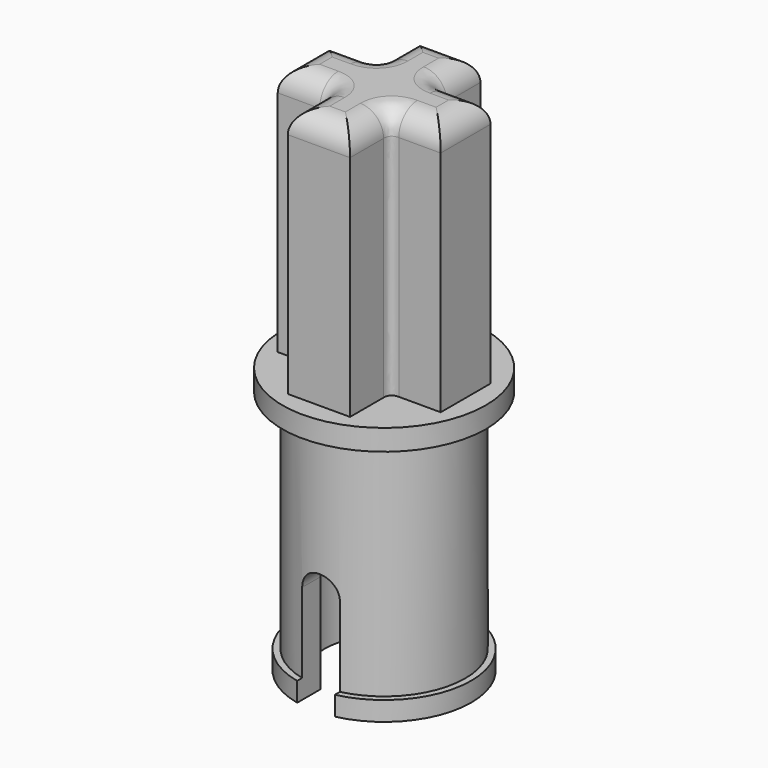
from build123d import *

# Parameters (mm, degrees)
F0_R         = 2.3495
F1_DEPTH     = 15.6718
F3_R         = 2.5273
F4_DEPTH     = 0.5588
F5_DEPTH     = 12.7
F6_R         = 2.9464
F7_DEPTH     = 8.5598
F8_R         = 12.7
F9_DEPTH     = 7.9502
F10_W        = 1.4605
F10_H        = 1.8034
F10_W_2      = 1.8034
F10_H_2      = 1.4605
F11_DEPTH    = 7.2898
F12_T1_DEPTH = 7.9030102448
F13_R        = 0.6745312693
F14_R        = 1.7145
F15_DEPTH    = 5.8674


# Not quite as in the source:
# - a fillet or chamfer that OpenCascade refuses, or shapes differently, is made with other operations: its cross-section is extruded or revolved along the edge and cut away or added


with BuildPart() as f1:
    # F0 (on Top) → F1 (new body)
    with BuildSketch(Plane.XY):
        Circle(F0_R)
    extrude(amount=F1_DEPTH)

    # F3 (on face) → F4 (join)
    with BuildSketch(Plane(origin=(0, 0, 0), x_dir=(1, 0, 0), z_dir=(0, 0, -1))):
        Circle(F3_R)
    extrude(amount=-F4_DEPTH)

    # F2 (on Front) → F5 (cut, symmetric)
    with BuildSketch(Plane.XZ):
        with BuildLine():
            Line((-0.5461, -2.8702), (0.5461, -2.8702))
            Line((0.5461, -2.8702), (0.5461, 2.8702))
            ThreePointArc((0.5461, 2.8702), (0, 2.3241), (-0.5461, 2.8702))
            Line((-0.5461, 2.8702), (-0.5461, -2.8702))
        make_face()
        with BuildLine():
            ThreePointArc((-0.5461, 2.8702), (0, 2.3241), (0.5461, 2.8702))
            Line((0.5461, 2.8702), (-0.5461, 2.8702))
        make_face()
        with BuildLine():
            Line((-0.5461, 2.8702), (0.5461, 2.8702))
            ThreePointArc((0.5461, 2.8702), (0, 3.4163), (-0.5461, 2.8702))
        make_face()
    extrude(amount=F5_DEPTH, both=True, mode=Mode.SUBTRACT)

    # F6 (on face) → F7 (join)
    with BuildSketch(Plane.XY.offset(15.6718)):
        Circle(F6_R)
    extrude(amount=-F7_DEPTH)

    # F8 (on face) → F9 (cut)
    with BuildSketch(Plane.XY.offset(15.6718)):
        Circle(F8_R)
    extrude(amount=-F9_DEPTH, mode=Mode.SUBTRACT)

    # F10 (on face) → F11 (join)
    with BuildSketch(Plane.XY.offset(7.7216)):
        with Locations((1.63195, 0)):
            Rectangle(F10_W, F10_H)
        with Locations((0, -1.63195)):
            Rectangle(F10_W_2, F10_H_2)
        Rectangle(F10_W_2, F10_H)
        with Locations((-1.63195, 0)):
            Rectangle(F10_W, F10_H)
        with Locations((0, 1.63195)):
            Rectangle(F10_W_2, F10_H_2)
    extrude(amount=F11_DEPTH)

    # F12: fillet of radius 0.2452840979 on 4 edges, made by hand

    # F12_s2 → F12_t1 (join)
    with BuildSketch(Plane.XY.offset(7.1083897552)):
        with BuildLine():
            add(Edge.make_bspline(
                [(-1.1469840979, -0.9017), (-0.9017, -0.9017), (-0.9017, -1.1469840979)],
                knots=[0, 0, 0, 1, 1, 1], degree=2, weights=[1, 1, 1]))
            Line((-0.9017, -1.1469840979), (-0.9017, -0.9017))
            Line((-0.9017, -0.9017), (-1.1469840979, -0.9017))
        make_face()
        with BuildLine():
            add(Edge.make_bspline(
                [(1.1469840979, 0.9017), (0.9017, 0.9017), (0.9017, 1.1469840979)],
                knots=[0, 0, 0, 1, 1, 1], degree=2, weights=[1, 1, 1]))
            Line((0.9017, 1.1469840979), (0.9017, 0.9017))
            Line((0.9017, 0.9017), (1.1469840979, 0.9017))
        make_face()
        with BuildLine():
            add(Edge.make_bspline(
                [(1.1469840979, -0.9017), (0.9017, -0.9017), (0.9017, -1.1469840979)],
                knots=[0, 0, 0, 1, 1, 1], degree=2, weights=[1, 1, 1]))
            Line((0.9017, -1.1469840979), (0.9017, -0.9017))
            Line((0.9017, -0.9017), (1.1469840979, -0.9017))
        make_face()
        with BuildLine():
            add(Edge.make_bspline(
                [(-0.9017, 1.1469840979), (-0.9017, 0.9017), (-1.1469840979, 0.9017)],
                knots=[0, 0, 0, 1, 1, 1], degree=2, weights=[1, 1, 1]))
            Line((-1.1469840979, 0.9017), (-0.9017, 0.9017))
            Line((-0.9017, 0.9017), (-0.9017, 1.1469840979))
        make_face()
    extrude(amount=F12_T1_DEPTH)

    # F13
    f13_edges = [f1.edges().sort_by_distance(p)[0] for p in [
        (1.754592, -0.9017, 15.0114),
        (2.3622, 0, 15.0114),
        (1.754592, 0.9017, 15.0114),
        (0.963022, 0.96302, 15.0114),
        (0.9017, 1.754592, 15.0114),
        (0, 2.3622, 15.0114),
        (-0.9017, 1.754592, 15.0114),
        (-0.96302, 0.963022, 15.0114),
        (-1.754592, 0.9017, 15.0114),
        (-2.3622, 0, 15.0114),
        (-1.754592, -0.9017, 15.0114),
        (-0.963022, -0.96302, 15.0114),
        (-0.9017, -1.754592, 15.0114),
        (0, -2.3622, 15.0114),
        (0.9017, -1.754592, 15.0114),
        (0.963022, -0.96302, 15.0114),
    ]]
    fillet(f13_edges, radius=F13_R)

    # F14 (on face) → F15 (cut)
    with BuildSketch(Plane(origin=(0, 0, 0), x_dir=(1, 0, 0), z_dir=(0, 0, -1))):
        Circle(F14_R)
    extrude(amount=-F15_DEPTH, mode=Mode.SUBTRACT)


solid = f1.part
